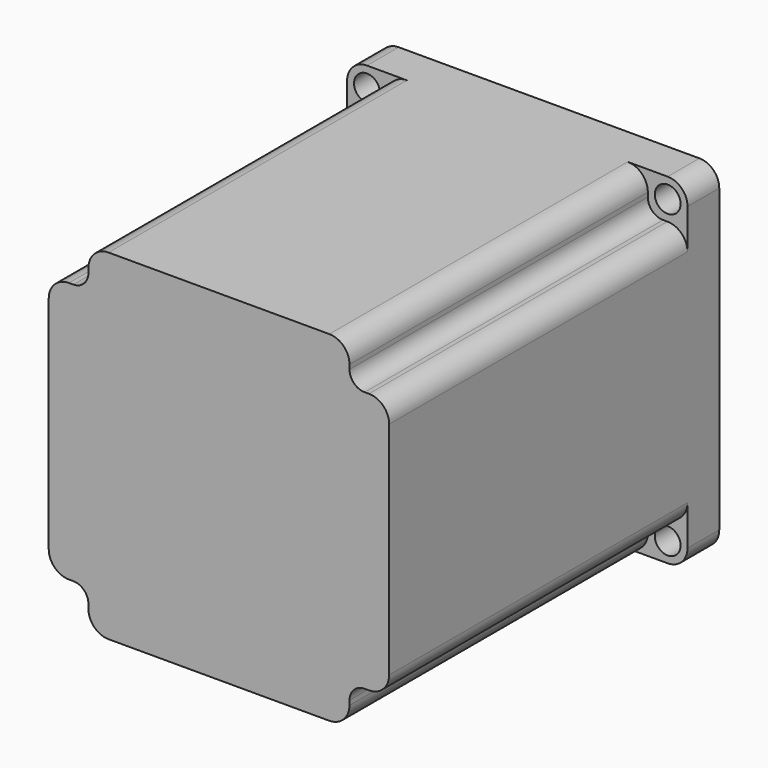
from build123d import *

# Parameters (mm, degrees)
F0_R     = 19.05
F0_R_2   = 3.25
F0_R_3   = 7
F1_DEPTH = 10
F3_DEPTH = 104
F4_R     = 5.08
F5_R     = 7
F6_DEPTH = 34
F7_R     = 19.05
F7_R_2   = 7
F8_DEPTH = 1.6


# Not quite as in the source:
# - a feature of the source that left no trace in its solid (it failed there, or was rolled back) is left out


with BuildPart() as f1:
    # F0 (on Front) → F1 (new body)
    with BuildSketch(Plane.XZ):
        Polygon((-32.9, -42.9), (32.9, -42.9), (32.9, -32.9), (42.9, -32.9), (42.9, 32.9), (32.9, 32.9), (32.9, 42.9), (-32.9, 42.9), (-32.9, 32.9), (-42.9, 32.9), (-42.9, -32.9), (-32.9, -32.9), align=None)
        Circle(F0_R, mode=Mode.SUBTRACT)
        with BuildLine():
            Line((-42.9, 37.9), (-42.9, 32.9))
            Line((-42.9, 32.9), (-32.9, 32.9))
            Line((-32.9, 32.9), (-32.9, 42.9))
            Line((-32.9, 42.9), (-37.9, 42.9))
            ThreePointArc((-37.9, 42.9), (-41.4355339059, 41.4355339059), (-42.9, 37.9))
        make_face()
        with Locations((-37.9, 37.9)):
            Circle(F0_R_2, mode=Mode.SUBTRACT)
        with BuildLine():
            Line((32.9, 32.9), (42.9, 32.9))
            Line((42.9, 32.9), (42.9, 37.9))
            ThreePointArc((42.9, 37.9), (41.4355339059, 41.4355339059), (37.9, 42.9))
            Line((37.9, 42.9), (32.9, 42.9))
            Line((32.9, 42.9), (32.9, 32.9))
        make_face()
        with Locations((37.9, 37.9)):
            Circle(F0_R_2, mode=Mode.SUBTRACT)
        Circle(F0_R)
        Circle(F0_R_3, mode=Mode.SUBTRACT)
        Circle(F0_R_3)
        with BuildLine():
            Line((-37.9, -42.9), (-32.9, -42.9))
            Line((-32.9, -42.9), (-32.9, -32.9))
            Line((-32.9, -32.9), (-42.9, -32.9))
            Line((-42.9, -32.9), (-42.9, -37.9))
            ThreePointArc((-42.9, -37.9), (-41.4344223535, -41.4344223535), (-37.9, -42.9))
        make_face()
        with Locations((-37.9, -37.9)):
            Circle(F0_R_2, mode=Mode.SUBTRACT)
        with BuildLine():
            Line((32.9, -42.9), (37.9, -42.9))
            ThreePointArc((37.9, -42.9), (41.4344223535, -41.4344223535), (42.9, -37.9))
            Line((42.9, -37.9), (42.9, -32.9))
            Line((42.9, -32.9), (32.9, -32.9))
            Line((32.9, -32.9), (32.9, -42.9))
        make_face()
        with Locations((37.9, -37.9)):
            Circle(F0_R_2, mode=Mode.SUBTRACT)
    extrude(amount=-F1_DEPTH)

    # F2 (on face) → F3 (join)
    with BuildSketch(Plane(origin=(0, 10, 0), x_dir=(-1, 0, 0), z_dir=(0, 1, 0))):
        with BuildLine():
            Line((32.9, 42.9), (-32.9, 42.9))
            Line((-32.9, 42.9), (-32.9, 36.71))
            ThreePointArc((-32.9, 36.71), (-34.0159231637, 34.0159231637), (-36.71, 32.9))
            Line((-36.71, 32.9), (-42.9, 32.9))
            Line((-42.9, 32.9), (-42.9, -32.9))
            Line((-42.9, -32.9), (-36.71, -32.9))
            ThreePointArc((-36.71, -32.9), (-34.0159231637, -34.0159231637), (-32.9, -36.71))
            Line((-32.9, -36.71), (-32.9, -42.9))
            Line((-32.9, -42.9), (32.9, -42.9))
            Line((32.9, -42.9), (32.9, -36.71))
            ThreePointArc((32.9, -36.71), (34.0159231637, -34.0159231637), (36.71, -32.9))
            Line((36.71, -32.9), (42.9, -32.9))
            Line((42.9, -32.9), (42.9, 32.9))
            Line((42.9, 32.9), (36.71, 32.9))
            ThreePointArc((36.71, 32.9), (34.0159231637, 34.0159231637), (32.9, 36.71))
            Line((32.9, 36.71), (32.9, 42.9))
        make_face()
    extrude(amount=-F3_DEPTH)

    # F4
    f4_edges = [f1.edges().sort_by_distance(p)[0] for p in [
        (-32.9, -47, 42.9),
        (32.9, -47, 42.9),
        (42.9, 5, 37.9),
        (-42.9, 5, 37.9),
        (-32.9, -47, -42.9),
        (32.9, -47, -42.9),
        (-42.9, -47, 32.9),
        (42.9, -47, -32.9),
        (42.9, -47, 32.9),
        (-42.9, -47, -32.9),
    ]]
    fillet(f4_edges, radius=F4_R)

    # F5 (on face) → F6 (join)
    with BuildSketch(Plane(origin=(0, 10, 0), x_dir=(-1, 0, 0), z_dir=(0, 1, 0))):
        Circle(F5_R)
    extrude(amount=F6_DEPTH)

    # F7 (on face) → F8 (join)
    with BuildSketch(Plane(origin=(0, 10, 0), x_dir=(-1, 0, 0), z_dir=(0, 1, 0))):
        Circle(F7_R)
        Circle(F7_R_2, mode=Mode.SUBTRACT)
    extrude(amount=F8_DEPTH)


solid = f1.part
